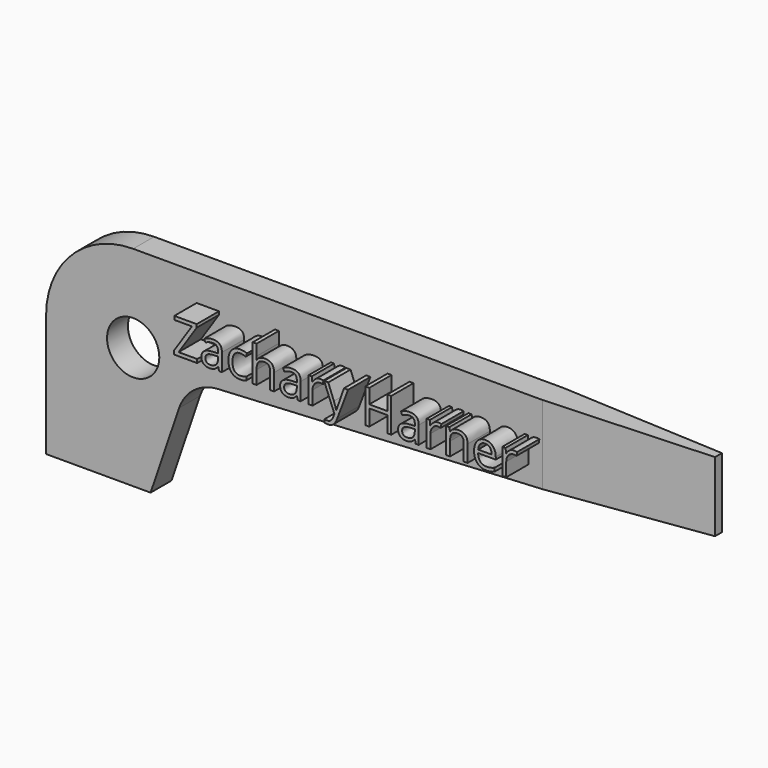
from build123d import *

# Parameters (mm, degrees)
F1_DEPTH     = 2.38125
F2_R         = 2.38125
F3_DEPTH     = 25.4
F5_DEPTH     = 25.4
F6_TEXT_SIZE = 4.3607957594
F7_DEPTH     = 2.54


# Not quite as in the source:
# - Text() gives the source's letters only with a copy of the font that has no kerning and outlines rounded to 1/6400 em; it was checked with that copy


with BuildPart() as f1:
    # F0 (on Front) → F1 (new body)
    with BuildSketch(Plane.XZ):
        with BuildLine():
            Line((60.325, 19.05), (7.9375, 19.05))
            ThreePointArc((7.9375, 19.05), (2.3248399243, 16.7251600757), (0, 11.1125))
            Line((0, 11.1125), (0, 0))
            Line((0, 0), (9.525, 0))
            Line((9.525, 0), (12.1173647876, 7.6271664624))
            ThreePointArc((12.1173647876, 7.6271664624), (13.4786145605, 9.5135918491), (15.6631963617, 10.3130942181))
            Line((15.6631963617, 10.3130942181), (60.325, 12.7))
            Line((60.325, 12.7), (60.325, 19.05))
        make_face()
    extrude(amount=F1_DEPTH)

    # F2 (on face) → F3 (cut)
    with BuildSketch(Plane.XZ.offset(2.38125)):
        with Locations((7.9375, 11.1125)):
            Circle(F2_R)
    extrude(amount=-F3_DEPTH, mode=Mode.SUBTRACT)

    # F4 (on face) → F5 (cut)
    with BuildSketch(Plane.XY.offset(19.05)):
        Polygon((60.325, 0), (45.24375, 0), (60.325, -0.79375), align=None)
        Polygon((60.325, -2.38125), (60.325, -1.5875), (45.24375, -2.38125), align=None)
    extrude(amount=-F5_DEPTH, mode=Mode.SUBTRACT)

    # F6 (on face) → F7 (join)
    with BuildSketch(Plane.XZ.offset(2.38125)):
        with Locations((13.49375, 13.4695567835)):
            Text('Zachary Harner', F6_TEXT_SIZE, font='Open Sans', text_align=(TextAlign.LEFT, TextAlign.BOTTOM))
    extrude(amount=F7_DEPTH)


solid = f1.part
